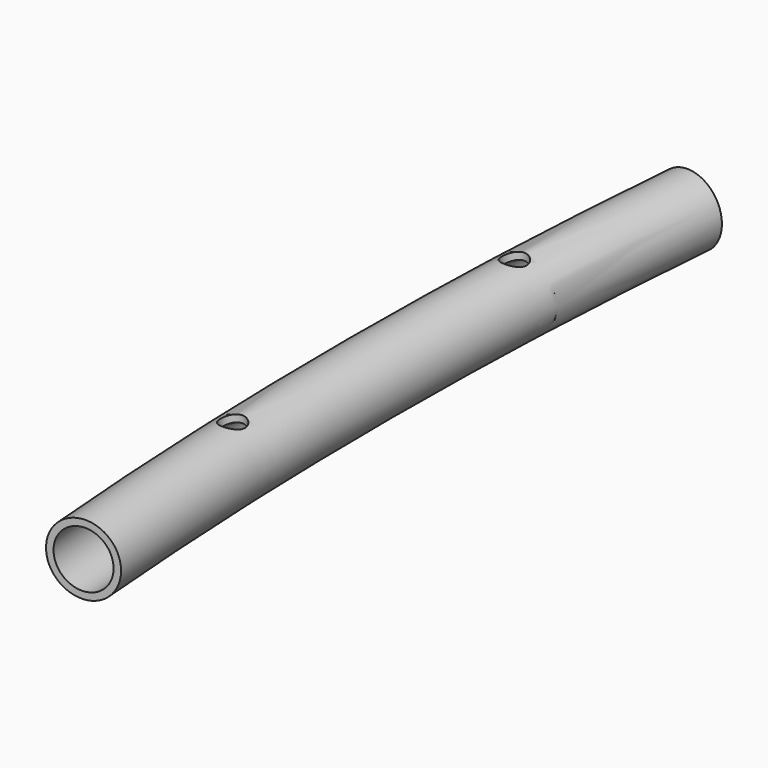
from build123d import *
from build123d import SkipClean  # not in build123d's __all__

# Parameters (mm, degrees)
F0_R          = 15
F0_R_2        = 12
F1_ANGLE_BACK = 5
F1_ANGLE      = 10
F2_R          = 5.25
F3_DEPTH      = 15.001
F3_DEPTH_BACK = 15.001


with BuildPart() as f1:
    # F0 (on Front) → F1 (revolve)
    with BuildSketch(Plane.XZ, mode=Mode.PRIVATE) as f1_sk:
        with Locations((-1850, 0)):
            Circle(F0_R)
        with Locations((-1850, 0)):
            Circle(F0_R_2, mode=Mode.SUBTRACT)
    revolve(f1_sk.sketch.rotate(Axis((0, 0, 190.0846064091), (0, 0, -1)), -F1_ANGLE_BACK), axis=Axis((0, 0, 190.0846064091), (0, 0, -1)), revolution_arc=F1_ANGLE)

    # F2 (on Top) → F3 (cut, two sides)
    with BuildSketch(Plane.XY) as f3_sk:
        with Locations((-1848.4791045614, -75)):
            Circle(F2_R)
        with Locations((-1848.4791045614, 75)):
            Circle(F2_R)
    with SkipClean():  # cleaning this boolean's faces spoils the solid; the shape is the same uncleaned
        extrude(amount=-F3_DEPTH, mode=Mode.SUBTRACT)
        extrude(f3_sk.sketch, amount=F3_DEPTH_BACK, mode=Mode.SUBTRACT)


solid = f1.part
